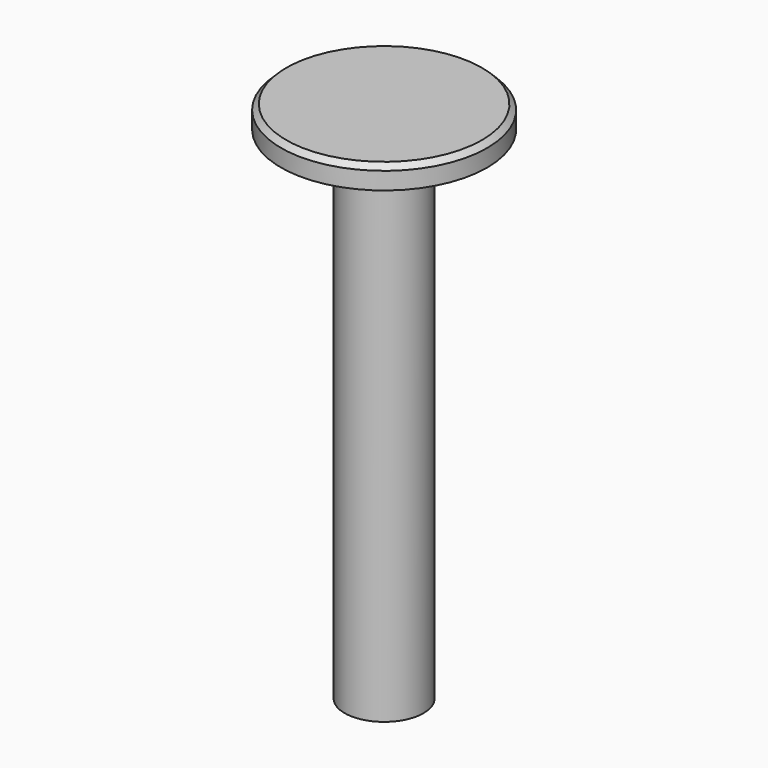
from build123d import *

# Parameters (mm, degrees)
F0_R      = 5.0038
F0_R_2    = 1.9145814382
F1_DEPTH  = 1.6002
F1_FACE_R = 5.0038
F2_DEPTH  = 0.508
F3_SIZE   = 0.254
F4_R      = 1.9145814382
F4_R_2    = 1.5836825197
F5_DEPTH  = 25.4


with BuildPart() as f1:
    # F0 (on Top) → F1 (new body)
    with BuildSketch(Plane.XY):
        Circle(F0_R)
        Circle(F0_R_2, mode=Mode.SUBTRACT)
        Circle(F0_R_2)
    extrude(amount=F1_DEPTH)

    # F0 (on Top) + F1_face (on face) → F2 (cut)
    with BuildSketch(Plane.XY):
        Circle(F0_R)
        Circle(F0_R_2, mode=Mode.SUBTRACT)
    with BuildSketch(Plane.XY.offset(1.6002)):
        Circle(F1_FACE_R)
    extrude(amount=-F2_DEPTH, mode=Mode.SUBTRACT)

    # F3
    f3_edges = [f1.edges().sort_by_distance(p)[0] for p in [
        (-5.0038, 0, 1.0922),
    ]]
    chamfer(f3_edges, length=F3_SIZE)

    # F4 (on face) → F5 (join)
    with BuildSketch(Plane.XY.offset(1.0922)):
        Circle(F4_R)
        Circle(F4_R_2, mode=Mode.SUBTRACT)
    extrude(amount=-F5_DEPTH)


solid = f1.part
